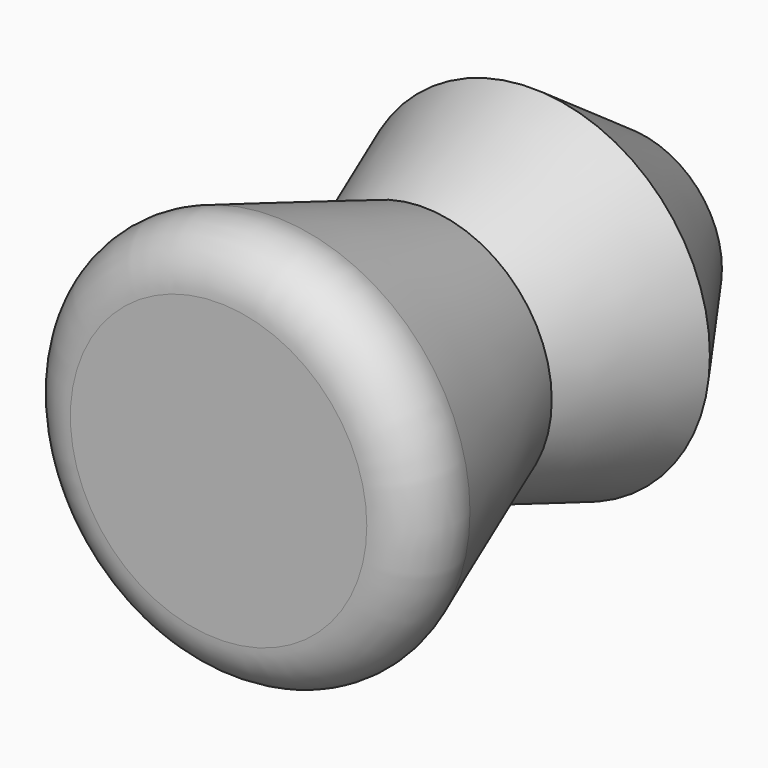
from build123d import *

# Parameters (mm, degrees)
F0_R     = 63.5
F1_DEPTH = 127
F1_TAPER = -20
F2_SIZE  = 63.5
F3_R     = 25.4


with BuildPart() as f1:
    # F0 (on Front) → F1 (new body, symmetric)
    with BuildSketch(Plane.XZ):
        Circle(F0_R)
    extrude(amount=F1_DEPTH, both=True, taper=F1_TAPER)

    # F2
    f2_edges = [f1.edges().sort_by_distance(p)[0] for p in [
        (-109.72422, 127, 0),
    ]]
    chamfer(f2_edges, length=F2_SIZE)

    # F3
    f3_edges = [f1.edges().sort_by_distance(p)[0] for p in [
        (-109.72422, -127, 0),
    ]]
    fillet(f3_edges, radius=F3_R)


solid = f1.part
